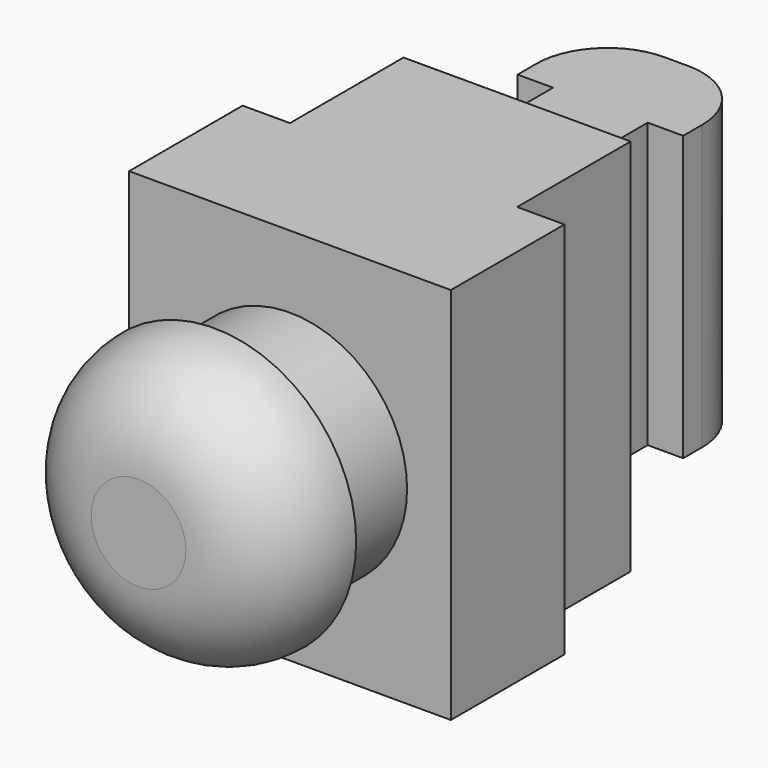
from build123d import *

# Parameters (mm, degrees)
F0_R      = 2.475
F1_DEPTH  = 2
F2_R      = 3
F3_DEPTH  = 2
F4_R      = 1.99999
F5_W      = 6.8
F5_H      = 8
F5_R      = 2.475
F6_DEPTH  = 3
F7_W      = 4.8
F7_H      = 8
F8_DEPTH  = 3
F9_W      = 2
F9_H      = 6
F10_DEPTH = 2.2
F11_W     = 0.75
F11_H     = 6
F11_W_2   = 2
F12_DEPTH = 2
F13_R     = 1.5


# Not quite as in the source:
# - a fillet or chamfer is up to 0.001 mm smaller than in the source, because OpenCascade refuses the exact size


with BuildPart() as f1:
    # F0 (on Front) → F1 (new body)
    with BuildSketch(Plane.XZ):
        Circle(F0_R)
    extrude(amount=F1_DEPTH)

    # F2 (on face) → F3 (join)
    with BuildSketch(Plane.XZ.offset(2)):
        Circle(F2_R)
    extrude(amount=F3_DEPTH)

    # F4 (radius 2 in the source; OpenCascade refuses exactly that, so slightly less here)
    f4_edges = [f1.edges().sort_by_distance(p)[0] for p in [
        (-3, -4, 0),
    ]]
    fillet(f4_edges, radius=F4_R)

    # F5 (on face) → F6 (join)
    with BuildSketch(Plane(origin=(0, 0, 0), x_dir=(-1, 0, 0), z_dir=(0, 1, 0))):
        Rectangle(F5_W, F5_H)
        Circle(F5_R, mode=Mode.SUBTRACT)
        Circle(F5_R)
    extrude(amount=F6_DEPTH)

    # F7 (on face) → F8 (join)
    with BuildSketch(Plane(origin=(0, 3, 0), x_dir=(-1, 0, 0), z_dir=(0, 1, 0))):
        Rectangle(F7_W, F7_H)
    extrude(amount=F8_DEPTH)

    # F9 (on face) → F10 (join)
    with BuildSketch(Plane(origin=(0, 6, 0), x_dir=(-1, 0, 0), z_dir=(0, 1, 0))):
        Rectangle(F9_W, F9_H)
    extrude(amount=F10_DEPTH)

    # F11 (on face) → F12 (join)
    with BuildSketch(Plane(origin=(0, 8.2, 0), x_dir=(-1, 0, 0), z_dir=(0, 1, 0))):
        with Locations((-1.375, 0)):
            Rectangle(F11_W, F11_H)
        Rectangle(F11_W_2, F11_H)
        with Locations((1.375, 0)):
            Rectangle(F11_W, F11_H)
    extrude(amount=F12_DEPTH)

    # F13
    f13_edges = [f1.edges().sort_by_distance(p)[0] for p in [
        (1.75, 10.2, 0),
        (-1.75, 10.2, 0),
    ]]
    fillet(f13_edges, radius=F13_R)


solid = f1.part
